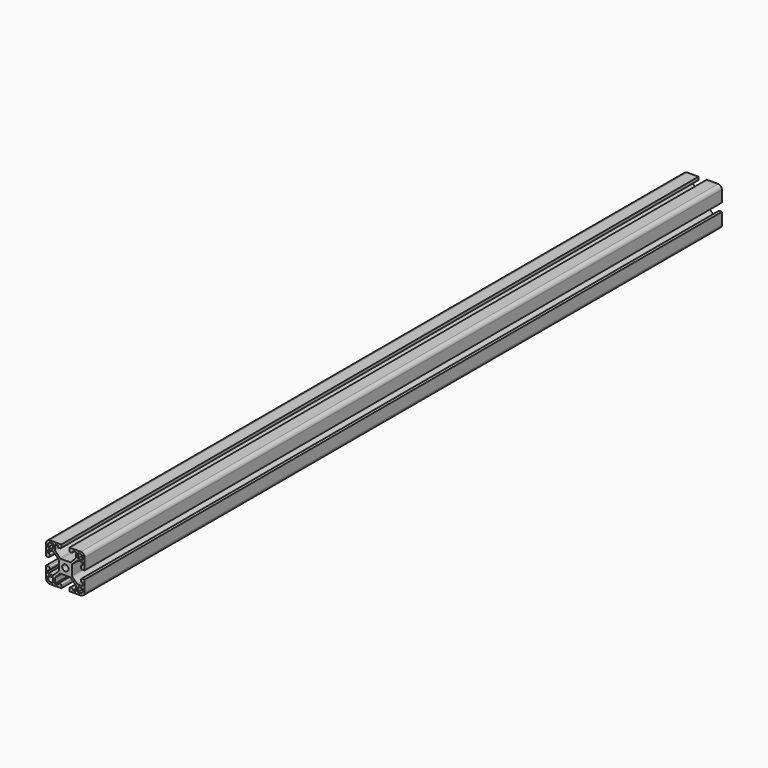
from build123d import *

# Parameters (mm, degrees)
F0_R     = 2.45
F1_DEPTH = 460
F2_DEPTH = 160


# Not quite as in the source:
# - ends of sketch curves that miss each other by under 0.0002 mm in the source are joined


with BuildPart() as f1:
    # F0 (on Front) → F1 (new body)
    with BuildSketch(Plane.XZ):
        with BuildLine():
            Line((-3.1749674082, 15), (-12, 15))
            ThreePointArc((-12, 15), (-14.1213203436, 14.1213203436), (-15, 12))
            Line((-15, 12), (-15, 3.175))
            Line((-15, 3.175), (-13.0855346263, 3.175))
            ThreePointArc((-13.0855346263, 3.175), (-12.3835980145, 3.4627605788), (-12.0856407741, 4.1604300138))
            Line((-12.0856407741, 4.1604300138), (-12.0761692778, 4.8104300138))
            ThreePointArc((-12.0761692778, 4.8104300138), (-12.3638237087, 5.5269366118), (-13.0760631299, 5.825))
            Line((-13.0760631299, 5.825), (-13.5, 5.825))
            Line((-13.5, 5.825), (-13.5, 8.225))
            Line((-13.5, 8.225), (-9.8968845016, 8.225))
            ThreePointArc((-9.8968845016, 8.225), (-9.5279915195, 8.1544718757), (-9.2111331975, 7.9528359354))
            Line((-9.2111331975, 7.9528359354), (-5.4142486959, 4.3754933338))
            ThreePointArc((-5.4142486959, 4.3754933338), (-5.1819174045, 4.0440465354), (-5.1, 3.6476573984))
            Line((-5.1, 3.6476573984), (-5.1, -3.4999243287))
            ThreePointArc((-5.1, -3.4999243287), (-5.1782354607, -3.8876744211), (-5.4007002683, -4.2147528992))
            Line((-5.4007002683, -4.2147528992), (-9.2084959767, -7.9398285705))
            ThreePointArc((-9.2084959767, -7.9398285705), (-9.5301904718, -8.1509666761), (-9.9077957084, -8.225))
            Line((-9.9077957084, -8.225), (-13.5, -8.225))
            Line((-13.5, -8.225), (-13.5, -5.825))
            Line((-13.5, -5.825), (-13.0760631299, -5.825))
            ThreePointArc((-13.0760631299, -5.825), (-12.3638237087, -5.5269366118), (-12.0761692778, -4.8104300138))
            Line((-12.0761692778, -4.8104300138), (-12.0856407741, -4.1604300138))
            ThreePointArc((-12.0856407741, -4.1604300138), (-12.3835980145, -3.4627605788), (-13.0855346263, -3.175))
            Line((-13.0855346263, -3.175), (-15, -3.175))
            Line((-15, -3.175), (-15, -12))
            ThreePointArc((-15, -12), (-14.1213203436, -14.1213203436), (-12, -15))
            Line((-12, -15), (-3.175, -15))
            Line((-3.175, -15), (-3.175, -13.0855346263))
            ThreePointArc((-3.175, -13.0855346263), (-3.4627605788, -12.3835980145), (-4.1604300138, -12.0856407741))
            Line((-4.1604300138, -12.0856407741), (-4.8104300138, -12.0761692778))
            ThreePointArc((-4.8104300138, -12.0761692778), (-5.5269366118, -12.3638237087), (-5.825, -13.0760631299))
            Line((-5.825, -13.0760631299), (-5.825, -13.5))
            Line((-5.825, -13.5), (-8.225, -13.5))
            Line((-8.225, -13.5), (-8.225, -9.8968845016))
            ThreePointArc((-8.225, -9.8968845016), (-8.1544718757, -9.5279915195), (-7.9528359354, -9.2111331975))
            Line((-7.9528359354, -9.2111331975), (-4.3754933338, -5.4142486959))
            ThreePointArc((-4.3754933338, -5.4142486959), (-4.0440465354, -5.1819174045), (-3.6476573984, -5.1))
            Line((-3.6476573984, -5.1), (3.4999243287, -5.1))
            ThreePointArc((3.4999243287, -5.1), (3.8876744211, -5.1782354607), (4.2147528992, -5.4007002683))
            Line((4.2147528992, -5.4007002683), (7.9398285705, -9.2084959767))
            ThreePointArc((7.9398285705, -9.2084959767), (8.1509666761, -9.5301904718), (8.225, -9.9077957084))
            Line((8.225, -9.9077957084), (8.225, -13.5))
            Line((8.225, -13.5), (5.825, -13.5))
            Line((5.825, -13.5), (5.825, -13.0760631299))
            ThreePointArc((5.825, -13.0760631299), (5.5269366118, -12.3638237087), (4.8104300138, -12.0761692778))
            Line((4.8104300138, -12.0761692778), (4.1604300138, -12.0856407741))
            ThreePointArc((4.1604300138, -12.0856407741), (3.4627605788, -12.3835980145), (3.175, -13.0855346263))
            Line((3.175, -13.0855346263), (3.175, -15))
            Line((3.175, -15), (12, -15))
            ThreePointArc((12, -15), (14.1213203436, -14.1213203436), (15, -12))
            Line((15, -12), (15, -3.175))
            Line((15, -3.175), (13.0855346263, -3.175))
            ThreePointArc((13.0855346263, -3.175), (12.3835980145, -3.4627605788), (12.0856407741, -4.1604300138))
            Line((12.0856407741, -4.1604300138), (12.0761692778, -4.8104300138))
            ThreePointArc((12.0761692778, -4.8104300138), (12.3638237087, -5.5269366118), (13.0760631299, -5.825))
            Line((13.0760631299, -5.825), (13.5, -5.825))
            Line((13.5, -5.825), (13.5, -8.225))
            Line((13.5, -8.225), (9.9077957084, -8.225))
            ThreePointArc((9.9077957084, -8.225), (9.5301904718, -8.1509666761), (9.2084959767, -7.9398285705))
            Line((9.2084959767, -7.9398285705), (5.4007002683, -4.2147528992))
            ThreePointArc((5.4007002683, -4.2147528992), (5.1782354607, -3.8876744211), (5.1, -3.4999243287))
            Line((5.1, -3.4999243287), (5.1, 3.6476573984))
            ThreePointArc((5.1, 3.6476573984), (5.1819174045, 4.0440465354), (5.4142486959, 4.3754933338))
            Line((5.4142486959, 4.3754933338), (9.2111331975, 7.9528359354))
            ThreePointArc((9.2111331975, 7.9528359354), (9.5279915195, 8.1544718757), (9.8968845016, 8.225))
            Line((9.8968845016, 8.225), (13.5, 8.225))
            Line((13.5, 8.225), (13.5, 5.825))
            Line((13.5, 5.825), (13.0760631299, 5.825))
            ThreePointArc((13.0760631299, 5.825), (12.3638237087, 5.5269366118), (12.0761692778, 4.8104300138))
            Line((12.0761692778, 4.8104300138), (12.0856407741, 4.1604300138))
            ThreePointArc((12.0856407741, 4.1604300138), (12.3835980145, 3.4627605788), (13.0855346263, 3.175))
            Line((13.0855346263, 3.175), (15, 3.175))
            Line((15, 3.175), (15, 12))
            ThreePointArc((15, 12), (14.1213203436, 14.1213203436), (12, 15))
            Line((12, 15), (3.1750325918, 15))
            Line((3.1750325918, 15), (3.1750325918, 13.0854824722))
            ThreePointArc((3.1750325918, 13.0854824722), (3.4627931706, 12.3835458604), (4.1604626057, 12.0855886201))
            Line((4.1604626057, 12.0855886201), (4.8104626057, 12.0761171237))
            ThreePointArc((4.8104626057, 12.0761171237), (5.5269692036, 12.3637715546), (5.8250325918, 13.0760109758))
            Line((5.8250325918, 13.0760109758), (5.8250325918, 13.4999478459))
            Line((5.8250325918, 13.4999478459), (8.2250325918, 13.4999478459))
            Line((8.2250325918, 13.4999478459), (8.2250325918, 9.8968323476))
            ThreePointArc((8.2250325918, 9.8968323476), (8.1545044675, 9.5279393654), (7.9528685272, 9.2110810434))
            Line((7.9528685272, 9.2110810434), (4.3755259256, 5.4141965418))
            ThreePointArc((4.3755259256, 5.4141965418), (4.0440791272, 5.1818652505), (3.6476899902, 5.0999478459))
            Line((3.6476899902, 5.0999478459), (-3.4998917369, 5.0999478459))
            ThreePointArc((-3.4998917369, 5.0999478459), (-3.8876418293, 5.1781833067), (-4.2147203074, 5.4006481142))
            Line((-4.2147203074, 5.4006481142), (-7.9397959787, 9.2084438226))
            ThreePointArc((-7.9397959787, 9.2084438226), (-8.1509340843, 9.5301383177), (-8.2249674082, 9.9077435543))
            Line((-8.2249674082, 9.9077435543), (-8.2249674082, 13.4999478459))
            Line((-8.2249674082, 13.4999478459), (-5.8249674082, 13.4999478459))
            Line((-5.8249674082, 13.4999478459), (-5.8249674082, 13.0760109758))
            ThreePointArc((-5.8249674082, 13.0760109758), (-5.5269040199, 12.3637715546), (-4.810397422, 12.0761171237))
            Line((-4.810397422, 12.0761171237), (-4.160397422, 12.0855886201))
            ThreePointArc((-4.160397422, 12.0855886201), (-3.462727987, 12.3835458604), (-3.1749674082, 13.0854824722))
            Line((-3.1749674082, 13.0854824722), (-3.1749674082, 15))
        make_face()
        with BuildLine():
            Line((-13.5, -11.5), (-13.5, -9.7))
            Line((-13.5, -9.7), (-9.7, -9.7))
            Line((-9.7, -9.7), (-9.7, -13.5))
            Line((-9.7, -13.5), (-11.5, -13.5))
            ThreePointArc((-11.5, -13.5), (-12.9142135624, -12.9142135624), (-13.5, -11.5))
        make_face(mode=Mode.SUBTRACT)
        with BuildLine():
            Line((9.7, -9.7), (13.5, -9.7))
            Line((13.5, -9.7), (13.5, -11.5))
            ThreePointArc((13.5, -11.5), (12.9142135624, -12.9142135624), (11.5, -13.5))
            Line((11.5, -13.5), (9.7, -13.5))
            Line((9.7, -13.5), (9.7, -9.7))
        make_face(mode=Mode.SUBTRACT)
        with BuildLine():
            ThreePointArc((-13.5, 11.5), (-12.9142135624, 12.9142135624), (-11.5, 13.5))
            Line((-11.5, 13.5), (-9.7, 13.5))
            Line((-9.7, 13.5), (-9.7, 9.7))
            Line((-9.7, 9.7), (-13.5, 9.7))
            Line((-13.5, 9.7), (-13.5, 11.5))
        make_face(mode=Mode.SUBTRACT)
        Circle(F0_R, mode=Mode.SUBTRACT)
        with BuildLine():
            Line((9.7, 13.5), (11.5, 13.5))
            ThreePointArc((11.5, 13.5), (12.9142135624, 12.9142135624), (13.5, 11.5))
            Line((13.5, 11.5), (13.5, 9.7))
            Line((13.5, 9.7), (9.7, 9.7))
            Line((9.7, 9.7), (9.7, 13.5))
        make_face(mode=Mode.SUBTRACT)
    extrude(amount=F1_DEPTH)

    # F2 (add): a face of the model
    f2_faces = [f1.faces().sort_by_distance(p)[0] for p in [
        (5.2291627207, -460, 12.6659491494),
    ]]
    extrude(f2_faces, amount=F2_DEPTH)


solid = f1.part
